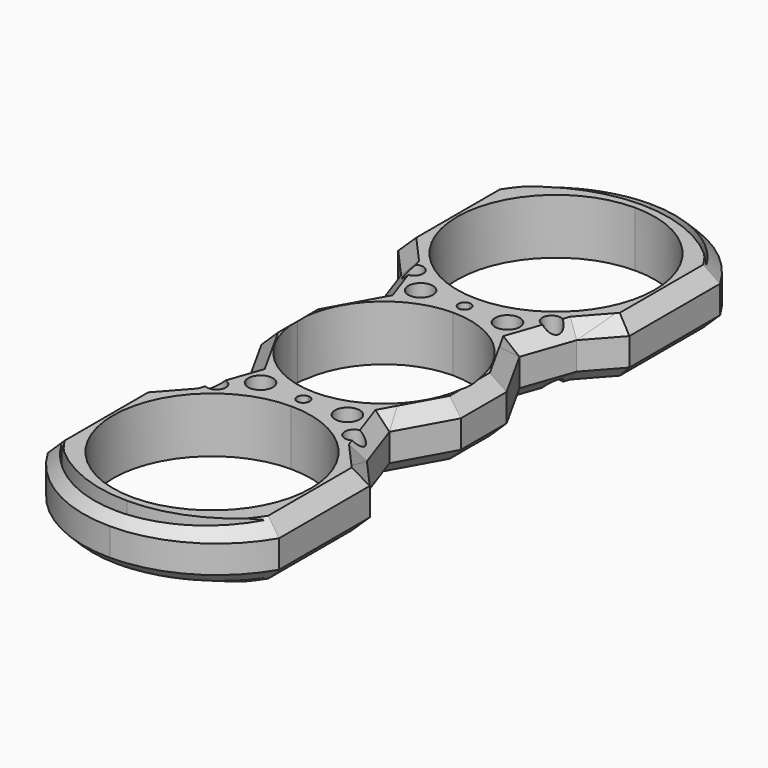
from build123d import *

# Parameters (mm, degrees)
F0_R          = 1.1983069663
F0_R_2        = 1.5880389974
F1_DEPTH      = 7.112
F2_T1_DEPTH   = 23.7091133916
F2_T3_DEPTH   = 16.4988505075
F2_T5_DEPTH   = 23.7091133916
F2_T8_ANGLE   = 171.8914289594
F2_T12_DEPTH  = 14.5046253488
F2_T17_DEPTH  = 15.930394403
F2_T23_DEPTH  = 16.8819871554
F2_T28_DEPTH  = 15.930394403
F2_T34_DEPTH  = 14.5046253488
F2_T39_DEPTH  = 16.8819871554
F2_T44_DEPTH  = 16.8819871554
F2_T49_DEPTH  = 15.930394403
F2_T55_DEPTH  = 14.5046253488
F2_T60_DEPTH  = 15.930394403
F2_T66_DEPTH  = 16.8819871554
F2_T71_DEPTH  = 14.5046253488
F2_T74_ANGLE  = 171.8914289594
F2_T76_ANGLE  = 171.8914289594
F2_T80_DEPTH  = 14.5046253488
F2_T85_DEPTH  = 15.930394403
F2_T91_DEPTH  = 16.8819871554
F2_T96_DEPTH  = 16.8819871554
F2_T101_DEPTH = 15.930394403
F2_T107_DEPTH = 14.5046253488
F2_T110_ANGLE = 171.8914289594
F2_T114_DEPTH = 14.5046253488
F2_T119_DEPTH = 15.930394403
F2_T125_DEPTH = 16.8819871554
F2_T130_DEPTH = 16.8819871554
F2_T135_DEPTH = 15.930394403
F2_T141_DEPTH = 14.5046253488


# Not quite as in the source:
# - a fillet or chamfer that OpenCascade refuses, or shapes differently, is made with other operations: its cross-section is extruded or revolved along the edge and cut away or added


with BuildPart() as f1:
    # F0 (on Top) → F1 (new body)
    with BuildSketch(Plane.XY):
        with BuildLine():
            ThreePointArc((-11.1125, 0), (-7.8577241059, 7.8577241059), (0, 11.1125))
            Line((0, 11.1125), (0, 12.1447060873))
            ThreePointArc((0, 12.1447060873), (-0.8062227945, 12.9509288818), (0, 13.7571516763))
            Line((0, 13.7571516763), (0, 14.9225))
            ThreePointArc((0, 14.9225), (-12.7, 27.6225), (0, 40.3225))
            Line((0, 40.3225), (0, 41.2482666662))
            ThreePointArc((0, 41.2482666662), (-7.2912161288, 39.6690625696), (-13.2735492662, 35.2117754519))
            ThreePointArc((-13.2735492662, 35.2117754519), (-7.6418208999, 40.7562008644), (0, 42.7710435083))
            Line((0, 42.7710435083), (0, 43.9781881869))
            ThreePointArc((0, 43.9781881869), (-8.5719346951, 41.6828182712), (-14.8497745395, 35.4110151529))
            Line((-14.8497745395, 35.4110151529), (-14.8497745395, 20.8468064666))
            Line((-14.8497745395, 20.8468064666), (-11.280115461, 16.848789528))
            Line((-11.280115461, 16.848789528), (-9.0495523811, 10.4403998094))
            Line((-9.0495523811, 10.4403998094), (-12.8070118018, 3.6769729012))
            Line((-12.8070118018, 3.6769729012), (-12.8070118018, 0))
            Line((-12.8070118018, 0), (-11.1125, 0))
        make_face()
        with Locations((-8.8490322232, 15.8545169979)):
            Circle(F0_R, mode=Mode.SUBTRACT)
        with Locations((-5.5815395899, 12.8507725894)):
            Circle(F0_R_2, mode=Mode.SUBTRACT)
        with BuildLine():
            ThreePointArc((0, 11.1125), (7.8577241059, 7.8577241059), (11.1125, 0))
            Line((11.1125, 0), (12.8070118018, 0))
            Line((12.8070118018, 0), (12.8070118018, 3.6769729012))
            Line((12.8070118018, 3.6769729012), (9.0495523811, 10.4403998094))
            Line((9.0495523811, 10.4403998094), (11.280115461, 16.848789528))
            Line((11.280115461, 16.848789528), (14.8497745395, 20.8468064666))
            Line((14.8497745395, 20.8468064666), (14.8497745395, 35.4110151529))
            ThreePointArc((14.8497745395, 35.4110151529), (8.5719346951, 41.6828182712), (0, 43.9781881869))
            Line((0, 43.9781881869), (0, 42.7710435083))
            ThreePointArc((0, 42.7710435083), (7.5041442912, 40.7975038507), (13.0891939625, 35.4110151529))
            ThreePointArc((13.0891939625, 35.4110151529), (7.1655527313, 39.7220445495), (0, 41.2482666662))
            Line((0, 41.2482666662), (0, 40.3225))
            ThreePointArc((0, 40.3225), (8.9802561211, 36.6027561211), (12.7, 27.6225))
            ThreePointArc((12.7, 27.6225), (8.9802561211, 18.6422438789), (0, 14.9225))
            Line((0, 14.9225), (0, 13.7571516763))
            ThreePointArc((0, 13.7571516763), (0.5700856051, 13.5210144869), (0.8062227945, 12.9509288818))
            ThreePointArc((0.8062227945, 12.9509288818), (0.5700856051, 12.3808432766), (0, 12.1447060873))
            Line((0, 12.1447060873), (0, 11.1125))
        make_face()
        with Locations((5.5815395899, 12.8507725894)):
            Circle(F0_R_2, mode=Mode.SUBTRACT)
        with Locations((8.8490322232, 15.8545169979)):
            Circle(F0_R, mode=Mode.SUBTRACT)
        with BuildLine():
            Line((0, -12.1447060873), (0, -11.1125))
            ThreePointArc((0, -11.1125), (-7.8577241059, -7.8577241059), (-11.1125, 0))
            Line((-11.1125, 0), (-12.8070118018, 0))
            Line((-12.8070118018, 0), (-12.8070118018, -3.6769729012))
            Line((-12.8070118018, -3.6769729012), (-9.0495523811, -10.4403998094))
            Line((-9.0495523811, -10.4403998094), (-11.280115461, -16.848789528))
            Line((-11.280115461, -16.848789528), (-14.8497745395, -20.8468064666))
            Line((-14.8497745395, -20.8468064666), (-14.8497745395, -35.4110151529))
            ThreePointArc((-14.8497745395, -35.4110151529), (-8.5719346951, -41.6828182712), (0, -43.9781881869))
            Line((0, -43.9781881869), (0, -42.7710435083))
            ThreePointArc((0, -42.7710435083), (-7.6418208999, -40.7562008644), (-13.2735492662, -35.2117754519))
            ThreePointArc((-13.2735492662, -35.2117754519), (-7.2912161288, -39.6690625696), (0, -41.2482666662))
            Line((0, -41.2482666662), (0, -40.3225))
            ThreePointArc((0, -40.3225), (-12.7, -27.6225), (0, -14.9225))
            Line((0, -14.9225), (0, -13.7571516763))
            ThreePointArc((0, -13.7571516763), (-0.8062227945, -12.9509288818), (0, -12.1447060873))
        make_face()
        with Locations((-8.8490322232, -15.8545169979)):
            Circle(F0_R, mode=Mode.SUBTRACT)
        with Locations((-5.5815395899, -12.8507725894)):
            Circle(F0_R_2, mode=Mode.SUBTRACT)
        with BuildLine():
            Line((12.8070118018, 0), (11.1125, 0))
            ThreePointArc((11.1125, 0), (7.8577241059, -7.8577241059), (0, -11.1125))
            Line((0, -11.1125), (0, -12.1447060873))
            ThreePointArc((0, -12.1447060873), (0.5700856051, -12.3808432766), (0.8062227945, -12.9509288818))
            ThreePointArc((0.8062227945, -12.9509288818), (0.5700856051, -13.5210144869), (0, -13.7571516763))
            Line((0, -13.7571516763), (0, -14.9225))
            ThreePointArc((0, -14.9225), (8.9802561211, -18.6422438789), (12.7, -27.6225))
            ThreePointArc((12.7, -27.6225), (8.9802561211, -36.6027561211), (0, -40.3225))
            Line((0, -40.3225), (0, -41.2482666662))
            ThreePointArc((0, -41.2482666662), (7.1655527313, -39.7220445495), (13.0891939625, -35.4110151529))
            ThreePointArc((13.0891939625, -35.4110151529), (7.5041442912, -40.7975038507), (0, -42.7710435083))
            Line((0, -42.7710435083), (0, -43.9781881869))
            ThreePointArc((0, -43.9781881869), (8.5719346951, -41.6828182712), (14.8497745395, -35.4110151529))
            Line((14.8497745395, -35.4110151529), (14.8497745395, -20.8468064666))
            Line((14.8497745395, -20.8468064666), (11.280115461, -16.848789528))
            Line((11.280115461, -16.848789528), (9.0495523811, -10.4403998094))
            Line((9.0495523811, -10.4403998094), (12.8070118018, -3.6769729012))
            Line((12.8070118018, -3.6769729012), (12.8070118018, 0))
        make_face()
        with Locations((5.5815395899, -12.8507725894)):
            Circle(F0_R_2, mode=Mode.SUBTRACT)
        with Locations((8.8490322232, -15.8545169979)):
            Circle(F0_R, mode=Mode.SUBTRACT)
    extrude(amount=F1_DEPTH)

    # F2: chamfer of 1.778 on 40 edges, made by hand

    # F2_s2 → F2_t1 (cut)
    with BuildSketch(Plane.XZ.offset(-39.9834675055)):
        Polygon((-14.8497745395, 5.334), (-13.0717745395, 7.112), (-14.8497745395, 7.112), align=None)
        Polygon((14.8497745395, 5.334), (13.0717745395, 7.112), (14.8497745395, 7.112), align=None)
        Polygon((14.8497745395, 1.778), (13.0717745395, 0), (14.8497745395, 0), align=None)
        Polygon((-14.8497745395, 1.778), (-13.0717745395, 0), (-14.8497745395, 0), align=None)
    extrude(amount=F2_T1_DEPTH, mode=Mode.SUBTRACT)

    # F2_s4 → F2_t3 (cut)
    with BuildSketch(Plane.XZ.offset(-8.2494252538)):
        Polygon((12.8070118018, 5.334), (11.0290118018, 7.112), (12.8070118018, 7.112), align=None)
        Polygon((-12.8070118018, 5.334), (-11.0290118018, 7.112), (-12.8070118018, 7.112), align=None)
        Polygon((-12.8070118018, 1.778), (-11.0290118018, 0), (-12.8070118018, 0), align=None)
        Polygon((12.8070118018, 1.778), (11.0290118018, 0), (12.8070118018, 0), align=None)
    extrude(amount=F2_T3_DEPTH, mode=Mode.SUBTRACT)

    # F2_s6 → F2_t5 (cut)
    with BuildSketch(Plane.XZ.offset(16.274354114)):
        Polygon((-14.8497745395, 5.334), (-13.0717745395, 7.112), (-14.8497745395, 7.112), align=None)
        Polygon((14.8497745395, 5.334), (13.0717745395, 7.112), (14.8497745395, 7.112), align=None)
        Polygon((-14.8497745395, 1.778), (-13.0717745395, 0), (-14.8497745395, 0), align=None)
        Polygon((14.8497745395, 1.778), (13.0717745395, 0), (14.8497745395, 0), align=None)
    extrude(amount=F2_T5_DEPTH, mode=Mode.SUBTRACT)

    # F2_s7 → F2_t8 (revolve, cut)
    with BuildSketch(Plane(origin=(-1.8918093526, 26.6907006845, 0), x_dir=(0, 0, 1), z_dir=(0.0707015954, -0.997497511, 0))):
        Polygon((5.334, -19.0499534674), (7.112, -17.2719534674), (7.112, -19.0499534674), align=None)
    revolve(axis=Axis((0, 26.8247901814, 7.112), (0, 0, 1)), revolution_arc=F2_T8_ANGLE, mode=Mode.SUBTRACT)


with BuildPart() as f2_tool10:
    # F2_s11 → F2_t12 (new body)
    with BuildSketch(Plane(origin=(-19.989170673, 22.3878642697, 0), x_dir=(0, 0, 1), z_dir=(0.6660158833, -0.7459375599, 0))):
        Polygon((5.334, -2.8072996372), (7.112, -4.5852996372), (7.112, -2.8072996372), align=None)
    extrude(amount=F2_T12_DEPTH)

    split(bisect_by=Plane(origin=(-4.9339638716, -1.7173608555, 5.2243016561), x_dir=(0.328725439, -0.9444255321, 0), z_dir=(-0.6678096981, -0.2324439871, 0.7071067812)), keep=Keep.TOP)


with BuildPart() as f1_1:
    add(f1.part)

    # F2_t9: cut F2_tool10
    add(f2_tool10.part, mode=Mode.SUBTRACT)


with BuildPart() as f2_tool15:
    # F2_s16 → F2_t17 (new body)
    with BuildSketch(Plane(origin=(-7.9528349133, 22.8484304935, 0), x_dir=(0, 0, 1), z_dir=(0.328725439, -0.9444255321, 0))):
        Polygon((5.334, 5.1146033122), (7.112, 3.3366033122), (7.112, 5.1146033122), align=None)
    extrude(amount=F2_T17_DEPTH)

    split(bisect_by=Plane(origin=(-8.0051120438, 4.447284501, 9.1575192201), x_dir=(-0.4856429339, -0.8741572746, 0), z_dir=(-0.6181225367, 0.3434014118, 0.7071067812)), keep=Keep.TOP)

    split(bisect_by=Plane(origin=(-0.9423803516, -0.8414112869, 1.2633501814), x_dir=(0.6660158833, -0.7459375599, 0), z_dir=(-0.5274575069, -0.4709443474, 0.7071067812)), keep=Keep.TOP)


with BuildPart() as f1_2:
    add(f1_1.part)

    # F2_t14: cut F2_tool15
    add(f2_tool15.part, mode=Mode.SUBTRACT)


with BuildPart() as f2_tool21:
    # F2_s22 → F2_t23 (new body)
    with BuildSketch(Plane(origin=(4.5184959792, 8.1332927035, 0), x_dir=(0, 0, 1), z_dir=(-0.4856429339, -0.8741572746, 0))):
        Polygon((5.334, 12.9810384403), (7.112, 11.2030384403), (7.112, 12.9810384403), align=None)
    extrude(amount=F2_T23_DEPTH)

    split(bisect_by=Plane(origin=(-4.9339638716, -1.7173608555, 5.2243016561), x_dir=(0.328725439, -0.9444255321, 0), z_dir=(-0.6678096981, -0.2324439871, 0.7071067812)), keep=Keep.TOP)


with BuildPart() as f1_3:
    add(f1_2.part)

    # F2_t20: cut F2_tool21
    add(f2_tool21.part, mode=Mode.SUBTRACT)


with BuildPart() as f2_tool26:
    # F2_s27 → F2_t28 (new body)
    with BuildSketch(Plane(origin=(2.7161090194, 7.8033592824, 0), x_dir=(0, 0, 1), z_dir=(0.328725439, 0.9444255321, 0))):
        Polygon((5.334, 5.1146033122), (7.112, 3.3366033122), (7.112, 5.1146033122), align=None)
    extrude(amount=F2_T28_DEPTH)

    split(bisect_by=Plane(origin=(8.0051120438, 4.447284501, 9.1575192201), x_dir=(-0.4856429339, 0.8741572746, 0), z_dir=(0.6181225367, 0.3434014118, 0.7071067812)), keep=Keep.TOP)

    split(bisect_by=Plane(origin=(0.9423803516, -0.8414112869, 1.2633501814), x_dir=(0.6660158833, 0.7459375599, 0), z_dir=(0.5274575069, -0.4709443474, 0.7071067812)), keep=Keep.TOP)


with BuildPart() as f1_4:
    add(f1_3.part)

    # F2_t25: cut F2_tool26
    add(f2_tool26.part, mode=Mode.SUBTRACT)


with BuildPart() as f2_tool32:
    # F2_s33 → F2_t34 (new body)
    with BuildSketch(Plane(origin=(10.3288598099, 11.56831943, 0), x_dir=(0, 0, 1), z_dir=(0.6660158833, 0.7459375599, 0))):
        Polygon((5.334, -2.8072996372), (7.112, -4.5852996372), (7.112, -2.8072996372), align=None)
    extrude(amount=F2_T34_DEPTH)

    split(bisect_by=Plane(origin=(4.9339638716, -1.7173608555, 5.2243016561), x_dir=(0.328725439, 0.9444255321, 0), z_dir=(0.6678096981, -0.2324439871, 0.7071067812)), keep=Keep.TOP)


with BuildPart() as f1_5:
    add(f1_4.part)

    # F2_t31: cut F2_tool32
    add(f2_tool32.part, mode=Mode.SUBTRACT)


with BuildPart() as f2_tool37:
    # F2_s38 → F2_t39 (new body)
    with BuildSketch(Plane(origin=(3.6801217925, -6.6242191785, 0), x_dir=(0, 0, 1), z_dir=(-0.4856429339, 0.8741572746, 0))):
        Polygon((5.334, 12.9810384403), (7.112, 11.2030384403), (7.112, 12.9810384403), align=None)
    extrude(amount=F2_T39_DEPTH)

    split(bisect_by=Plane(origin=(4.9339638716, -1.7173608555, 5.2243016561), x_dir=(0.328725439, 0.9444255321, 0), z_dir=(0.6678096981, -0.2324439871, 0.7071067812)), keep=Keep.TOP)


with BuildPart() as f1_6:
    add(f1_5.part)

    # F2_t36: cut F2_tool37
    add(f2_tool37.part, mode=Mode.SUBTRACT)


with BuildPart() as f2_tool42:
    # F2_s43 → F2_t44 (new body)
    with BuildSketch(Plane(origin=(-3.6801217925, 6.6242191785, 0), x_dir=(0, 0, 1), z_dir=(0.4856429339, -0.8741572746, 0))):
        Polygon((5.334, 12.9810384403), (7.112, 11.2030384403), (7.112, 12.9810384403), align=None)
    extrude(amount=F2_T44_DEPTH)

    split(bisect_by=Plane(origin=(-4.9339638716, 1.7173608555, 5.2243016561), x_dir=(-0.328725439, -0.9444255321, 0), z_dir=(-0.6678096981, 0.2324439871, 0.7071067812)), keep=Keep.TOP)


with BuildPart() as f1_7:
    add(f1_6.part)

    # F2_t41: cut F2_tool42
    add(f2_tool42.part, mode=Mode.SUBTRACT)


with BuildPart() as f2_tool47:
    # F2_s48 → F2_t49 (new body)
    with BuildSketch(Plane(origin=(-2.7161090194, -7.8033592824, 0), x_dir=(0, 0, 1), z_dir=(-0.328725439, -0.9444255321, 0))):
        Polygon((5.334, 5.1146033122), (7.112, 3.3366033122), (7.112, 5.1146033122), align=None)
    extrude(amount=F2_T49_DEPTH)

    split(bisect_by=Plane(origin=(-0.9423803516, 0.8414112869, 1.2633501814), x_dir=(-0.6660158833, -0.7459375599, 0), z_dir=(-0.5274575069, 0.4709443474, 0.7071067812)), keep=Keep.TOP)

    split(bisect_by=Plane(origin=(-8.0051120438, -4.447284501, 9.1575192201), x_dir=(0.4856429339, -0.8741572746, 0), z_dir=(-0.6181225367, -0.3434014118, 0.7071067812)), keep=Keep.TOP)


with BuildPart() as f1_8:
    add(f1_7.part)

    # F2_t46: cut F2_tool47
    add(f2_tool47.part, mode=Mode.SUBTRACT)


with BuildPart() as f2_tool53:
    # F2_s54 → F2_t55 (new body)
    with BuildSketch(Plane(origin=(-10.3288598099, -11.56831943, 0), x_dir=(0, 0, 1), z_dir=(-0.6660158833, -0.7459375599, 0))):
        Polygon((5.334, -2.8072996372), (7.112, -4.5852996372), (7.112, -2.8072996372), align=None)
    extrude(amount=F2_T55_DEPTH)

    split(bisect_by=Plane(origin=(-4.9339638716, 1.7173608555, 5.2243016561), x_dir=(-0.328725439, -0.9444255321, 0), z_dir=(-0.6678096981, 0.2324439871, 0.7071067812)), keep=Keep.TOP)


with BuildPart() as f1_9:
    add(f1_8.part)

    # F2_t52: cut F2_tool53
    add(f2_tool53.part, mode=Mode.SUBTRACT)


with BuildPart() as f2_tool58:
    # F2_s59 → F2_t60 (new body)
    with BuildSketch(Plane(origin=(7.9528349133, -22.8484304935, 0), x_dir=(0, 0, 1), z_dir=(-0.328725439, 0.9444255321, 0))):
        Polygon((5.334, 5.1146033122), (7.112, 3.3366033122), (7.112, 5.1146033122), align=None)
    extrude(amount=F2_T60_DEPTH)

    split(bisect_by=Plane(origin=(8.0051120438, -4.447284501, 9.1575192201), x_dir=(0.4856429339, 0.8741572746, 0), z_dir=(0.6181225367, -0.3434014118, 0.7071067812)), keep=Keep.TOP)

    split(bisect_by=Plane(origin=(0.9423803516, 0.8414112869, 1.2633501814), x_dir=(-0.6660158833, 0.7459375599, 0), z_dir=(0.5274575069, 0.4709443474, 0.7071067812)), keep=Keep.TOP)


with BuildPart() as f1_10:
    add(f1_9.part)

    # F2_t57: cut F2_tool58
    add(f2_tool58.part, mode=Mode.SUBTRACT)


with BuildPart() as f2_tool64:
    # F2_s65 → F2_t66 (new body)
    with BuildSketch(Plane(origin=(-4.5184959792, -8.1332927035, 0), x_dir=(0, 0, 1), z_dir=(0.4856429339, 0.8741572746, 0))):
        Polygon((5.334, 12.9810384403), (7.112, 11.2030384403), (7.112, 12.9810384403), align=None)
    extrude(amount=F2_T66_DEPTH)

    split(bisect_by=Plane(origin=(4.9339638716, 1.7173608555, 5.2243016561), x_dir=(-0.328725439, 0.9444255321, 0), z_dir=(0.6678096981, 0.2324439871, 0.7071067812)), keep=Keep.TOP)


with BuildPart() as f1_11:
    add(f1_10.part)

    # F2_t63: cut F2_tool64
    add(f2_tool64.part, mode=Mode.SUBTRACT)


with BuildPart() as f2_tool69:
    # F2_s70 → F2_t71 (new body)
    with BuildSketch(Plane(origin=(19.989170673, -22.3878642697, 0), x_dir=(0, 0, 1), z_dir=(-0.6660158833, 0.7459375599, 0))):
        Polygon((5.334, -2.8072996372), (7.112, -4.5852996372), (7.112, -2.8072996372), align=None)
    extrude(amount=F2_T71_DEPTH)

    split(bisect_by=Plane(origin=(4.9339638716, 1.7173608555, 5.2243016561), x_dir=(-0.328725439, 0.9444255321, 0), z_dir=(0.6678096981, 0.2324439871, 0.7071067812)), keep=Keep.TOP)


with BuildPart() as f1_12:
    add(f1_11.part)

    # F2_t68: cut F2_tool69
    add(f2_tool69.part, mode=Mode.SUBTRACT)

    # F2_s73 → F2_t74 (revolve, cut)
    with BuildSketch(Plane(origin=(1.8918093526, -26.6907006845, 0), x_dir=(0, 0, 1), z_dir=(-0.0707015954, 0.997497511, 0))):
        Polygon((5.334, -19.0499534674), (7.112, -17.2719534674), (7.112, -19.0499534674), align=None)
    revolve(axis=Axis((0, -26.8247901814, 7.112), (0, 0, 1)), revolution_arc=F2_T74_ANGLE, mode=Mode.SUBTRACT)

    # F2_s75 → F2_t76 (revolve, cut)
    with BuildSketch(Plane(origin=(-1.8918093526, 26.6907006845, 0), x_dir=(0, 0, 1), z_dir=(0.0707015954, -0.997497511, 0))):
        Polygon((1.778, -19.0499534674), (0, -17.2719534674), (0, -19.0499534674), align=None)
    revolve(axis=Axis((0, 26.8247901814, 0), (0, 0, 1)), revolution_arc=F2_T76_ANGLE, mode=Mode.SUBTRACT)


with BuildPart() as f2_tool78:
    # F2_s79 → F2_t80 (new body)
    with BuildSketch(Plane(origin=(-19.989170673, 22.3878642697, 0), x_dir=(0, 0, 1), z_dir=(0.6660158833, -0.7459375599, 0))):
        Polygon((1.778, -2.8072996372), (0, -4.5852996372), (0, -2.8072996372), align=None)
    extrude(amount=F2_T80_DEPTH)

    split(bisect_by=Plane(origin=(-1.5755866793, -0.5484131943, -1.6683016561), x_dir=(0.328725439, -0.9444255321, 0), z_dir=(-0.6678096981, -0.2324439871, -0.7071067812)), keep=Keep.TOP)


with BuildPart() as f1_13:
    add(f1_12.part)

    # F2_t77: cut F2_tool78
    add(f2_tool78.part, mode=Mode.SUBTRACT)


with BuildPart() as f2_tool83:
    # F2_s84 → F2_t85 (new body)
    with BuildSketch(Plane(origin=(-7.9528349133, 22.8484304935, 0), x_dir=(0, 0, 1), z_dir=(0.328725439, -0.9444255321, 0))):
        Polygon((1.778, 5.1146033122), (0, 3.3366033122), (0, 5.1146033122), align=None)
    extrude(amount=F2_T85_DEPTH)

    split(bisect_by=Plane(origin=(-4.8966087752, 2.7203382282, -5.6015192201), x_dir=(-0.4856429339, -0.8741572746, 0), z_dir=(-0.6181225367, 0.3434014118, -0.7071067812)), keep=Keep.TOP)

    split(bisect_by=Plane(origin=(1.7101736114, 1.5269411939, 2.2926498186), x_dir=(0.6660158833, -0.7459375599, 0), z_dir=(-0.5274575069, -0.4709443474, -0.7071067812)), keep=Keep.TOP)


with BuildPart() as f1_14:
    add(f1_13.part)

    # F2_t82: cut F2_tool83
    add(f2_tool83.part, mode=Mode.SUBTRACT)


with BuildPart() as f2_tool89:
    # F2_s90 → F2_t91 (new body)
    with BuildSketch(Plane(origin=(4.5184959792, 8.1332927035, 0), x_dir=(0, 0, 1), z_dir=(-0.4856429339, -0.8741572746, 0))):
        Polygon((1.778, 12.9810384403), (0, 11.2030384403), (0, 12.9810384403), align=None)
    extrude(amount=F2_T91_DEPTH)

    split(bisect_by=Plane(origin=(-1.5755866793, -0.5484131943, -1.6683016561), x_dir=(0.328725439, -0.9444255321, 0), z_dir=(-0.6678096981, -0.2324439871, -0.7071067812)), keep=Keep.TOP)


with BuildPart() as f1_15:
    add(f1_14.part)

    # F2_t88: cut F2_tool89
    add(f2_tool89.part, mode=Mode.SUBTRACT)


with BuildPart() as f2_tool94:
    # F2_s95 → F2_t96 (new body)
    with BuildSketch(Plane(origin=(-3.6801217925, 6.6242191785, 0), x_dir=(0, 0, 1), z_dir=(0.4856429339, -0.8741572746, 0))):
        Polygon((1.778, 12.9810384403), (0, 11.2030384403), (0, 12.9810384403), align=None)
    extrude(amount=F2_T96_DEPTH)

    split(bisect_by=Plane(origin=(-1.5755866793, 0.5484131943, -1.6683016561), x_dir=(-0.328725439, -0.9444255321, 0), z_dir=(-0.6678096981, 0.2324439871, -0.7071067812)), keep=Keep.TOP)


with BuildPart() as f1_16:
    add(f1_15.part)

    # F2_t93: cut F2_tool94
    add(f2_tool94.part, mode=Mode.SUBTRACT)


with BuildPart() as f2_tool99:
    # F2_s100 → F2_t101 (new body)
    with BuildSketch(Plane(origin=(-2.7161090194, -7.8033592824, 0), x_dir=(0, 0, 1), z_dir=(-0.328725439, -0.9444255321, 0))):
        Polygon((1.778, 5.1146033122), (0, 3.3366033122), (0, 5.1146033122), align=None)
    extrude(amount=F2_T101_DEPTH)

    split(bisect_by=Plane(origin=(-4.8966087752, -2.7203382282, -5.6015192201), x_dir=(0.4856429339, -0.8741572746, 0), z_dir=(-0.6181225367, -0.3434014118, -0.7071067812)), keep=Keep.TOP)

    split(bisect_by=Plane(origin=(1.7101736114, -1.5269411939, 2.2926498186), x_dir=(-0.6660158833, -0.7459375599, 0), z_dir=(-0.5274575069, 0.4709443474, -0.7071067812)), keep=Keep.TOP)


with BuildPart() as f1_17:
    add(f1_16.part)

    # F2_t98: cut F2_tool99
    add(f2_tool99.part, mode=Mode.SUBTRACT)


with BuildPart() as f2_tool105:
    # F2_s106 → F2_t107 (new body)
    with BuildSketch(Plane(origin=(-10.3288598099, -11.56831943, 0), x_dir=(0, 0, 1), z_dir=(-0.6660158833, -0.7459375599, 0))):
        Polygon((1.778, -2.8072996372), (0, -4.5852996372), (0, -2.8072996372), align=None)
    extrude(amount=F2_T107_DEPTH)

    split(bisect_by=Plane(origin=(-1.5755866793, 0.5484131943, -1.6683016561), x_dir=(-0.328725439, -0.9444255321, 0), z_dir=(-0.6678096981, 0.2324439871, -0.7071067812)), keep=Keep.TOP)


with BuildPart() as f1_18:
    add(f1_17.part)

    # F2_t104: cut F2_tool105
    add(f2_tool105.part, mode=Mode.SUBTRACT)

    # F2_s109 → F2_t110 (revolve, cut)
    with BuildSketch(Plane(origin=(1.8918093526, -26.6907006845, 0), x_dir=(0, 0, 1), z_dir=(-0.0707015954, 0.997497511, 0))):
        Polygon((1.778, -19.0499534674), (0, -17.2719534674), (0, -19.0499534674), align=None)
    revolve(axis=Axis((0, -26.8247901814, 0), (0, 0, 1)), revolution_arc=F2_T110_ANGLE, mode=Mode.SUBTRACT)


with BuildPart() as f2_tool112:
    # F2_s113 → F2_t114 (new body)
    with BuildSketch(Plane(origin=(10.3288598099, 11.56831943, 0), x_dir=(0, 0, 1), z_dir=(0.6660158833, 0.7459375599, 0))):
        Polygon((1.778, -2.8072996372), (0, -4.5852996372), (0, -2.8072996372), align=None)
    extrude(amount=F2_T114_DEPTH)

    split(bisect_by=Plane(origin=(1.5755866793, -0.5484131943, -1.6683016561), x_dir=(0.328725439, 0.9444255321, 0), z_dir=(0.6678096981, -0.2324439871, -0.7071067812)), keep=Keep.TOP)


with BuildPart() as f1_19:
    add(f1_18.part)

    # F2_t111: cut F2_tool112
    add(f2_tool112.part, mode=Mode.SUBTRACT)


with BuildPart() as f2_tool117:
    # F2_s118 → F2_t119 (new body)
    with BuildSketch(Plane(origin=(2.7161090194, 7.8033592824, 0), x_dir=(0, 0, 1), z_dir=(0.328725439, 0.9444255321, 0))):
        Polygon((1.778, 5.1146033122), (0, 3.3366033122), (0, 5.1146033122), align=None)
    extrude(amount=F2_T119_DEPTH)

    split(bisect_by=Plane(origin=(-1.7101736114, 1.5269411939, 2.2926498186), x_dir=(0.6660158833, 0.7459375599, 0), z_dir=(0.5274575069, -0.4709443474, -0.7071067812)), keep=Keep.TOP)

    split(bisect_by=Plane(origin=(4.8966087752, 2.7203382282, -5.6015192201), x_dir=(-0.4856429339, 0.8741572746, 0), z_dir=(0.6181225367, 0.3434014118, -0.7071067812)), keep=Keep.TOP)


with BuildPart() as f1_20:
    add(f1_19.part)

    # F2_t116: cut F2_tool117
    add(f2_tool117.part, mode=Mode.SUBTRACT)


with BuildPart() as f2_tool123:
    # F2_s124 → F2_t125 (new body)
    with BuildSketch(Plane(origin=(3.6801217925, -6.6242191785, 0), x_dir=(0, 0, 1), z_dir=(-0.4856429339, 0.8741572746, 0))):
        Polygon((1.778, 12.9810384403), (0, 11.2030384403), (0, 12.9810384403), align=None)
    extrude(amount=F2_T125_DEPTH)

    split(bisect_by=Plane(origin=(1.5755866793, -0.5484131943, -1.6683016561), x_dir=(0.328725439, 0.9444255321, 0), z_dir=(0.6678096981, -0.2324439871, -0.7071067812)), keep=Keep.TOP)


with BuildPart() as f1_21:
    add(f1_20.part)

    # F2_t122: cut F2_tool123
    add(f2_tool123.part, mode=Mode.SUBTRACT)


with BuildPart() as f2_tool128:
    # F2_s129 → F2_t130 (new body)
    with BuildSketch(Plane(origin=(-4.5184959792, -8.1332927035, 0), x_dir=(0, 0, 1), z_dir=(0.4856429339, 0.8741572746, 0))):
        Polygon((1.778, 12.9810384403), (0, 11.2030384403), (0, 12.9810384403), align=None)
    extrude(amount=F2_T130_DEPTH)

    split(bisect_by=Plane(origin=(1.5755866793, 0.5484131943, -1.6683016561), x_dir=(-0.328725439, 0.9444255321, 0), z_dir=(0.6678096981, 0.2324439871, -0.7071067812)), keep=Keep.TOP)


with BuildPart() as f1_22:
    add(f1_21.part)

    # F2_t127: cut F2_tool128
    add(f2_tool128.part, mode=Mode.SUBTRACT)


with BuildPart() as f2_tool133:
    # F2_s134 → F2_t135 (new body)
    with BuildSketch(Plane(origin=(7.9528349133, -22.8484304935, 0), x_dir=(0, 0, 1), z_dir=(-0.328725439, 0.9444255321, 0))):
        Polygon((1.778, 5.1146033122), (0, 3.3366033122), (0, 5.1146033122), align=None)
    extrude(amount=F2_T135_DEPTH)

    split(bisect_by=Plane(origin=(4.8966087752, -2.7203382282, -5.6015192201), x_dir=(0.4856429339, 0.8741572746, 0), z_dir=(0.6181225367, -0.3434014118, -0.7071067812)), keep=Keep.TOP)

    split(bisect_by=Plane(origin=(-1.7101736114, -1.5269411939, 2.2926498186), x_dir=(-0.6660158833, 0.7459375599, 0), z_dir=(0.5274575069, 0.4709443474, -0.7071067812)), keep=Keep.TOP)


with BuildPart() as f1_23:
    add(f1_22.part)

    # F2_t132: cut F2_tool133
    add(f2_tool133.part, mode=Mode.SUBTRACT)


with BuildPart() as f2_tool139:
    # F2_s140 → F2_t141 (new body)
    with BuildSketch(Plane(origin=(19.989170673, -22.3878642697, 0), x_dir=(0, 0, 1), z_dir=(-0.6660158833, 0.7459375599, 0))):
        Polygon((1.778, -2.8072996372), (0, -4.5852996372), (0, -2.8072996372), align=None)
    extrude(amount=F2_T141_DEPTH)

    split(bisect_by=Plane(origin=(1.5755866793, 0.5484131943, -1.6683016561), x_dir=(-0.328725439, 0.9444255321, 0), z_dir=(0.6678096981, 0.2324439871, -0.7071067812)), keep=Keep.TOP)


with BuildPart() as f1_24:
    add(f1_23.part)

    # F2_t138: cut F2_tool139
    add(f2_tool139.part, mode=Mode.SUBTRACT)


solid = f1_24.part
